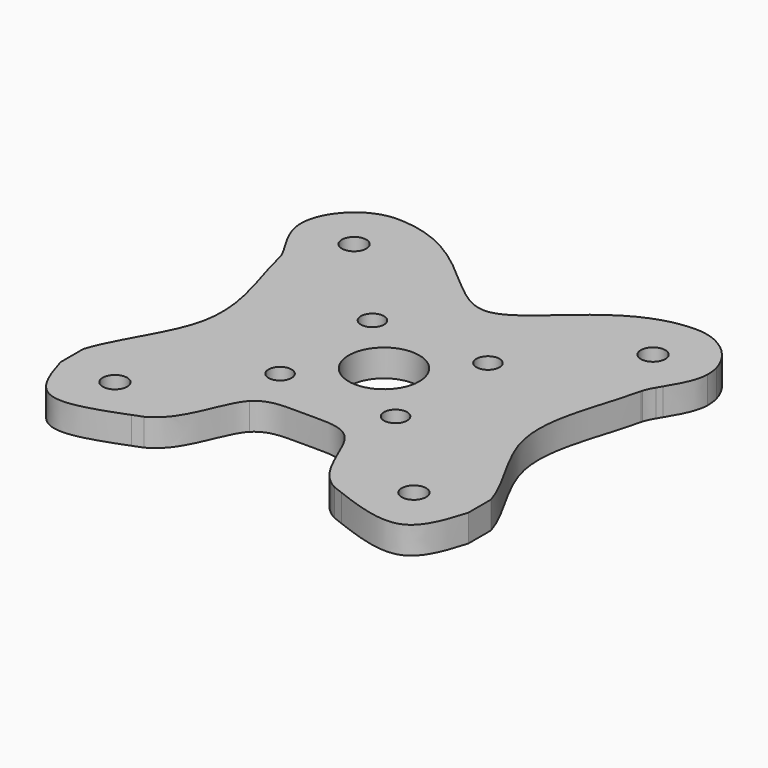
from build123d import *

# Parameters (mm, degrees)
F3_R     = 0.9
F3_R_2   = 0.85
F3_R_3   = 2.6
F4_DEPTH = 2


with BuildPart() as f4:
    # F3 (on offset) → F4 (new body)
    with BuildSketch(Plane.XY.offset(5)):
        with BuildLine():
            add(Edge.make_bspline(
                [(13.5840897294, 15.5610671266), (13.3511585546, 17.1029676873), (12.6074515763, 18.5088140753), (11, 19.5610671266)],
                knots=[0.7544415636, 0.7544415636, 0.7544415636, 0.7544415636, 0.7967305031, 0.7967305031, 0.7967305031, 0.7967305031], degree=3))
            ThreePointArc((11, 19.5610671266), (8.1715728753, 18.3894942513), (7, 15.5610671266))
            Line((7, 15.5610671266), (10.1, 15.5610671266))
            ThreePointArc((10.1, 15.5610671266), (11, 16.4610671266), (11.9, 15.5610671266))
            Line((11.9, 15.5610671266), (13.5840897294, 15.5610671266))
        make_face()
        with BuildLine():
            add(Edge.make_bspline(
                [(14.8754677726, 16.5513951244), (14.4362064353, 18.1121245067), (12.8992511156, 19.5610671266), (11, 19.5610671266)],
                knots=[0.5598679958, 0.5598679958, 0.5598679958, 0.5598679958, 1, 1, 1, 1], degree=3))
            add(Edge.make_bspline(
                [(13.5840897294, 15.5610671266), (13.3511585546, 17.1029676873), (12.6074515763, 18.5088140753), (11, 19.5610671266)],
                knots=[0.7544415636, 0.7544415636, 0.7544415636, 0.7544415636, 0.7967305031, 0.7967305031, 0.7967305031, 0.7967305031], degree=3))
            Line((13.5840897294, 15.5610671266), (15, 15.5610671266))
            ThreePointArc((15, 15.5610671266), (14.9687448325, 16.0601307044), (14.8754677726, 16.5513951244))
        make_face()
        with BuildLine():
            ThreePointArc((7, 15.5610671266), (8.1715728753, 18.3894942513), (11, 19.5610671266))
            add(Edge.make_bspline(
                [(3.1801327541, 15.5610671266), (5.1521059489, 17.258924835), (7.5281581703, 19.5610671266), (11, 19.5610671266)],
                knots=[0.6843780155, 0.6843780155, 0.6843780155, 0.6843780155, 1, 1, 1, 1], degree=3))
            Line((3.1801327541, 15.5610671266), (7, 15.5610671266))
        make_face()
        with BuildLine():
            add(Edge.make_bspline(
                [(-11, 19.5610671266), (-7.5281581703, 19.5610671266), (-5.1521059489, 17.258924835), (-3.1801327541, 15.5610671266)],
                knots=[0, 0, 0, 0, 0.3156219845, 0.3156219845, 0.3156219845, 0.3156219845], degree=3))
            add(Edge.make_bspline(
                [(-11, 19.5610671266), (-12.6074515763, 18.5088140753), (-13.3511585546, 17.1029676873), (-13.5840897294, 15.5610671266)],
                knots=[0.9225775171, 0.9225775171, 0.9225775171, 0.9225775171, 0.9648664566, 0.9648664566, 0.9648664566, 0.9648664566], degree=3))
            Line((-13.5840897294, 15.5610671266), (-11.9, 15.5610671266))
            ThreePointArc((-11.9, 15.5610671266), (-11, 16.4610671266), (-10.1, 15.5610671266))
            Line((-10.1, 15.5610671266), (-3.1801327541, 15.5610671266))
        make_face()
        with BuildLine():
            add(Edge.make_bspline(
                [(-11, 19.5610671266), (-12.6074515763, 18.5088140753), (-13.3511585546, 17.1029676873), (-13.5840897294, 15.5610671266)],
                knots=[0.9225775171, 0.9225775171, 0.9225775171, 0.9225775171, 0.9648664566, 0.9648664566, 0.9648664566, 0.9648664566], degree=3))
            add(Edge.make_bspline(
                [(-15, 15.7741791911), (-14.9345041339, 17.5934219618), (-13.2132485479, 19.5610671266), (-11, 19.5610671266)],
                knots=[0.4871023051, 0.4871023051, 0.4871023051, 0.4871023051, 1, 1, 1, 1], degree=3))
            Line((-15, 15.7741791911), (-15, 15.5610671266))
            Line((-15, 15.5610671266), (-13.5840897294, 15.5610671266))
        make_face()
        with BuildLine():
            Line((10.1, 15.5610671266), (7, 15.5610671266))
            ThreePointArc((7, 15.5610671266), (7.384697146, 13.8494639969), (8.4647926368, 12.4670852867))
            Line((8.4647926368, 12.4670852867), (13.4691565234, 12.4670852867))
            Line((13.4691565234, 12.4670852867), (13.492215644, 12.4670852867))
            add(Edge.make_bspline(
                [(13.492215644, 12.4670852867), (13.6721160747, 13.5160999102), (13.734281279, 14.5668660077), (13.5840897294, 15.5610671266)],
                knots=[0.7271741042, 0.7271741042, 0.7271741042, 0.7271741042, 0.7544415636, 0.7544415636, 0.7544415636, 0.7544415636], degree=3))
            Line((13.5840897294, 15.5610671266), (11.9, 15.5610671266))
            ThreePointArc((11.9, 15.5610671266), (11, 14.6610671266), (10.1, 15.5610671266))
        make_face()
        with BuildLine():
            ThreePointArc((8.4647926368, 12.4670852867), (7.384697146, 13.8494639969), (7, 15.5610671266))
            Line((7, 15.5610671266), (3.1801327541, 15.5610671266))
            add(Edge.make_bspline(
                [(-3.1801327541, 15.5610671266), (-2.0281581703, 14.5692235599), (0, 12.9979712148), (2.0281581703, 14.5692235599), (3.1801327541, 15.5610671266)],
                knots=[0.3156219845, 0.3156219845, 0.3156219845, 0.3156219845, 0.5, 0.6843780155, 0.6843780155, 0.6843780155, 0.6843780155], degree=3))
            Line((-3.1801327541, 15.5610671266), (-10.1, 15.5610671266))
            ThreePointArc((-10.1, 15.5610671266), (-11, 14.6610671266), (-11.9, 15.5610671266))
            Line((-11.9, 15.5610671266), (-13.5840897294, 15.5610671266))
            add(Edge.make_bspline(
                [(-13.5840897294, 15.5610671266), (-13.734281279, 14.5668660077), (-13.6721160747, 13.5160999102), (-13.492215644, 12.4670852867)],
                knots=[0.9648664566, 0.9648664566, 0.9648664566, 0.9648664566, 0.992133916, 0.992133916, 0.992133916, 0.992133916], degree=3))
            Line((-13.492215644, 12.4670852867), (-13.4691565234, 12.4670852867))
            Line((-13.4691565234, 12.4670852867), (8.4647926368, 12.4670852867))
        make_face()
        with BuildLine():
            Line((15, 15.5610671266), (13.5840897294, 15.5610671266))
            add(Edge.make_bspline(
                [(13.492215644, 12.4670852867), (13.6721160747, 13.5160999102), (13.734281279, 14.5668660077), (13.5840897294, 15.5610671266)],
                knots=[0.7271741042, 0.7271741042, 0.7271741042, 0.7271741042, 0.7544415636, 0.7544415636, 0.7544415636, 0.7544415636], degree=3))
            Line((13.492215644, 12.4670852867), (13.5352073632, 12.4670852867))
            ThreePointArc((13.5352073632, 12.4670852867), (13.7336426306, 12.6409304914), (13.9201867728, 12.8274780551))
            add(Edge.make_bspline(
                [(13.9201867728, 12.8274780551), (14.3914007653, 13.6110512692), (14.9629553276, 14.5497192982), (15, 15.5610671266)],
                knots=[0.1795179278, 0.1795179278, 0.1795179278, 0.1795179278, 0.4669985441, 0.4669985441, 0.4669985441, 0.4669985441], degree=3))
        make_face()
        with BuildLine():
            add(Edge.make_bspline(
                [(-13.5840897294, 15.5610671266), (-13.734281279, 14.5668660077), (-13.6721160747, 13.5160999102), (-13.492215644, 12.4670852867)],
                knots=[0.9648664566, 0.9648664566, 0.9648664566, 0.9648664566, 0.992133916, 0.992133916, 0.992133916, 0.992133916], degree=3))
            Line((-13.5840897294, 15.5610671266), (-15, 15.5610671266))
            add(Edge.make_bspline(
                [(-13.7063183417, 12.4670852867), (-14.1968968928, 13.3154705741), (-14.9570867675, 14.3895031275), (-15, 15.5610671266)],
                knots=[0.1339756897, 0.1339756897, 0.1339756897, 0.1339756897, 0.4669985441, 0.4669985441, 0.4669985441, 0.4669985441], degree=3))
            Line((-13.7063183417, 12.4670852867), (-13.492215644, 12.4670852867))
        make_face()
        with BuildLine():
            Line((13.4691565234, 12.4670852867), (8.4647926368, 12.4670852867))
            ThreePointArc((8.4647926368, 12.4670852867), (10.9507937826, 11.5613697945), (13.4583242546, 12.4056524377))
            Line((13.4583242546, 12.4056524377), (13.4691565234, 12.4670852867))
        make_face()
        with BuildLine():
            ThreePointArc((13.4583242546, 12.4056524377), (10.9507937826, 11.5613697945), (8.4647926368, 12.4670852867))
            Line((8.4647926368, 12.4670852867), (-13.4691565234, 12.4670852867))
            Line((-13.4691565234, 12.4670852867), (-13.3094010768, 11.5610671266))
            add(Edge.make_bspline(
                [(-13.3094010768, 11.5610671266), (-12.5871033108, 8.4210285266), (-9.9260749254, 3.2919220303), (-14.403876313, -2.3381175367), (-15, -4.3559935783)],
                knots=[0, 0, 0, 0, 0.0820790806, 0.1416655097, 0.1416655097, 0.1416655097, 0.1416655097], degree=3))
            Line((-15, -4.3559935783), (-15, -6.4389328734))
            add(Edge.make_bspline(
                [(-15, -6.4389328734), (-14.1595926628, -8.4371784368), (-10.2189124595, -9.723491879), (-7.7225640289, -9.0286027112)],
                knots=[0.1638195279, 0.1638195279, 0.1638195279, 0.1638195279, 0.2339911879, 0.2339911879, 0.2339911879, 0.2339911879], degree=3))
            add(Edge.make_bspline(
                [(-7.7225640289, -9.0286027112), (-7.4825681334, -8.9358330473), (-7.2413616339, -8.8417932594), (-7, -8.7483339502)],
                knots=[0.9423734081, 0.9423734081, 0.9423734081, 0.9423734081, 1, 1, 1, 1], degree=3))
            add(Edge.make_bspline(
                [(-7, -8.7483339502), (-4.9275830737, -7.6704662943), (-4.6345461271, -4.6287367083), (-3.5, -3.4389328734)],
                knots=[0.2412420108, 0.2412420108, 0.2412420108, 0.2412420108, 0.3089022709, 0.3089022709, 0.3089022709, 0.3089022709], degree=3))
            add(Edge.make_bspline(
                [(-3.5, -3.4389328734), (-2.6489806718, -2.5464649198), (0, -2.84548287), (2.6489806718, -2.5464649198), (3.5, -3.4389328734)],
                knots=[0.3089022709, 0.3089022709, 0.3089022709, 0.3089022709, 0.3596540101, 0.4104057492, 0.4104057492, 0.4104057492, 0.4104057492], degree=3))
            add(Edge.make_bspline(
                [(3.5, -3.4389328734), (4.6345461271, -4.6287367083), (4.9275830737, -7.6704662943), (7, -8.7483339502)],
                knots=[0.4104057492, 0.4104057492, 0.4104057492, 0.4104057492, 0.4780660094, 0.4780660094, 0.4780660094, 0.4780660094], degree=3))
            add(Edge.make_bspline(
                [(7.7349288931, -9.0320251809), (7.4908824059, -8.9385878573), (7.2455387097, -8.8434106938), (7, -8.7483339502)],
                knots=[0.9412809289, 0.9412809289, 0.9412809289, 0.9412809289, 1, 1, 1, 1], degree=3))
            add(Edge.make_bspline(
                [(7.7349288931, -9.0320251809), (10.2319042389, -9.7192464231), (14.1609789052, -8.4338823534), (15, -6.4389328734)],
                knots=[0.4854325797, 0.4854325797, 0.4854325797, 0.4854325797, 0.5554884923, 0.5554884923, 0.5554884923, 0.5554884923], degree=3))
            Line((15, -6.4389328734), (15, -4.3559935783))
            add(Edge.make_bspline(
                [(15, -4.3559935783), (14.403876313, -2.3381175367), (9.9260749254, 3.2919220303), (12.5871033108, 8.4210285266), (13.3094010768, 11.5610671266)],
                knots=[0.5776425105, 0.5776425105, 0.5776425105, 0.5776425105, 0.6372289396, 0.7193080202, 0.7193080202, 0.7193080202, 0.7193080202], degree=3))
            Line((13.3094010768, 11.5610671266), (13.4583242546, 12.4056524377))
        make_face()
        with Locations((-11, -6.4389328734)):
            Circle(F3_R, mode=Mode.SUBTRACT)
        with Locations((-4.25, 0.3110671266)):
            Circle(F3_R_2, mode=Mode.SUBTRACT)
        with Locations((0, 4.5610671266)):
            Circle(F3_R_3, mode=Mode.SUBTRACT)
        with Locations((11, -6.4389328734)):
            Circle(F3_R, mode=Mode.SUBTRACT)
        with Locations((4.25, 0.3110671266)):
            Circle(F3_R_2, mode=Mode.SUBTRACT)
        with Locations((-4.25, 8.8110671266)):
            Circle(F3_R_2, mode=Mode.SUBTRACT)
        with Locations((4.25, 8.8110671266)):
            Circle(F3_R_2, mode=Mode.SUBTRACT)
        with BuildLine():
            Line((13.5352073632, 12.4670852867), (13.492215644, 12.4670852867))
            add(Edge.make_bspline(
                [(13.4852520955, 12.4268172926), (13.4875924233, 12.4402395891), (13.4899136722, 12.4536622945), (13.492215644, 12.4670852867)],
                knots=[0.726825195, 0.726825195, 0.726825195, 0.726825195, 0.7271741042, 0.7271741042, 0.7271741042, 0.7271741042], degree=3))
            ThreePointArc((13.4852520955, 12.4268172926), (13.5103104732, 12.4468511212), (13.5352073632, 12.4670852867))
        make_face()
        with BuildLine():
            add(Edge.make_bspline(
                [(13.4852520955, 12.4268172926), (13.4875924233, 12.4402395891), (13.4899136722, 12.4536622945), (13.492215644, 12.4670852867)],
                knots=[0.726825195, 0.726825195, 0.726825195, 0.726825195, 0.7271741042, 0.7271741042, 0.7271741042, 0.7271741042], degree=3))
            Line((13.492215644, 12.4670852867), (13.4691565234, 12.4670852867))
            Line((13.4691565234, 12.4670852867), (13.4583242546, 12.4056524377))
            ThreePointArc((13.4583242546, 12.4056524377), (13.4718108282, 12.4162060438), (13.4852520955, 12.4268172926))
        make_face()
        with BuildLine():
            add(Edge.make_bspline(
                [(13.7063183417, 12.4670852867), (13.7734069659, 12.5831054462), (13.8455377753, 12.7033455891), (13.9201867728, 12.8274780551)],
                knots=[0.1339756897, 0.1339756897, 0.1339756897, 0.1339756897, 0.1795179278, 0.1795179278, 0.1795179278, 0.1795179278], degree=3))
            ThreePointArc((13.9201867728, 12.8274780551), (13.7336426306, 12.6409304914), (13.5352073632, 12.4670852867))
            Line((13.5352073632, 12.4670852867), (13.7063183417, 12.4670852867))
        make_face()
        with BuildLine():
            Line((-13.4691565234, 12.4670852867), (-13.492215644, 12.4670852867))
            add(Edge.make_bspline(
                [(-13.492215644, 12.4670852867), (-13.4466612755, 12.2014539119), (-13.3935576871, 11.9359348422), (-13.3344412049, 11.671474935)],
                knots=[0.992133916, 0.992133916, 0.992133916, 0.992133916, 0.9990385792, 0.9990385792, 0.9990385792, 0.9990385792], degree=3))
            add(Edge.make_bspline(
                [(-13.3094010768, 11.5610671266), (-13.3157403301, 11.597018819), (-13.324143718, 11.6338287797), (-13.3344412049, 11.671474935)],
                knots=[0, 0, 0, 0, 0.0185309619, 0.0185309619, 0.0185309619, 0.0185309619], degree=3))
            Line((-13.3094010768, 11.5610671266), (-13.4691565234, 12.4670852867))
        make_face()
        with BuildLine():
            add(Edge.make_bspline(
                [(-13.492215644, 12.4670852867), (-13.4466612755, 12.2014539119), (-13.3935576871, 11.9359348422), (-13.3344412049, 11.671474935)],
                knots=[0.992133916, 0.992133916, 0.992133916, 0.992133916, 0.9990385792, 0.9990385792, 0.9990385792, 0.9990385792], degree=3))
            Line((-13.492215644, 12.4670852867), (-13.7063183417, 12.4670852867))
            add(Edge.make_bspline(
                [(-13.3344412049, 11.671474935), (-13.3985927892, 11.9060040524), (-13.5362558173, 12.1729865265), (-13.7063183417, 12.4670852867)],
                knots=[0.0185309619, 0.0185309619, 0.0185309619, 0.0185309619, 0.1339756897, 0.1339756897, 0.1339756897, 0.1339756897], degree=3))
        make_face()
        with BuildLine():
            ThreePointArc((13.4852520955, 12.4268172926), (13.4718108282, 12.4162060438), (13.4583242546, 12.4056524377))
            Line((13.4583242546, 12.4056524377), (13.3094010768, 11.5610671266))
            add(Edge.make_bspline(
                [(13.3094010768, 11.5610671266), (13.3157403301, 11.597018819), (13.324143718, 11.6338287797), (13.3344412049, 11.671474935)],
                knots=[0, 0, 0, 0, 0.0185309619, 0.0185309619, 0.0185309619, 0.0185309619], degree=3))
            add(Edge.make_bspline(
                [(13.3344412049, 11.671474935), (13.390570389, 11.9225710471), (13.4412790174, 12.1746219822), (13.4852520955, 12.4268172926)],
                knots=[0.720269441, 0.720269441, 0.720269441, 0.720269441, 0.726825195, 0.726825195, 0.726825195, 0.726825195], degree=3))
        make_face()
        with BuildLine():
            ThreePointArc((13.5352073632, 12.4670852867), (13.5103104732, 12.4468511212), (13.4852520955, 12.4268172926))
            add(Edge.make_bspline(
                [(13.3344412049, 11.671474935), (13.390570389, 11.9225710471), (13.4412790174, 12.1746219822), (13.4852520955, 12.4268172926)],
                knots=[0.720269441, 0.720269441, 0.720269441, 0.720269441, 0.726825195, 0.726825195, 0.726825195, 0.726825195], degree=3))
            add(Edge.make_bspline(
                [(13.3344412049, 11.671474935), (13.3985927892, 11.9060040524), (13.5362558173, 12.1729865265), (13.7063183417, 12.4670852867)],
                knots=[0.0185309619, 0.0185309619, 0.0185309619, 0.0185309619, 0.1339756897, 0.1339756897, 0.1339756897, 0.1339756897], degree=3))
            Line((13.7063183417, 12.4670852867), (13.5352073632, 12.4670852867))
        make_face()
        with BuildLine():
            add(Edge.make_bspline(
                [(15, -6.4389328734), (14.55, -7.9389328734), (13.5150373015, -11.0782924932), (9.776904521, -9.8138300729), (7.7349288931, -9.0320251809)],
                knots=[0, 0, 0, 0, 0.4499691569, 0.9412809289, 0.9412809289, 0.9412809289, 0.9412809289], degree=3))
            add(Edge.make_bspline(
                [(7.7349288931, -9.0320251809), (10.2319042389, -9.7192464231), (14.1609789052, -8.4338823534), (15, -6.4389328734)],
                knots=[0.4854325797, 0.4854325797, 0.4854325797, 0.4854325797, 0.5554884923, 0.5554884923, 0.5554884923, 0.5554884923], degree=3))
        make_face()
        with BuildLine():
            add(Edge.make_bspline(
                [(-15, -6.4389328734), (-14.1595926628, -8.4371784368), (-10.2189124595, -9.723491879), (-7.7225640289, -9.0286027112)],
                knots=[0.1638195279, 0.1638195279, 0.1638195279, 0.1638195279, 0.2339911879, 0.2339911879, 0.2339911879, 0.2339911879], degree=3))
            add(Edge.make_bspline(
                [(-15, -6.4389328734), (-14.55, -7.9389328734), (-13.5253754228, -11.1597748555), (-9.7695536439, -9.8198601549), (-7.7225640289, -9.0286027112)],
                knots=[0, 0, 0, 0, 0.4508606887, 0.9423734081, 0.9423734081, 0.9423734081, 0.9423734081], degree=3))
        make_face()
    extrude(amount=F4_DEPTH)


solid = f4.part
